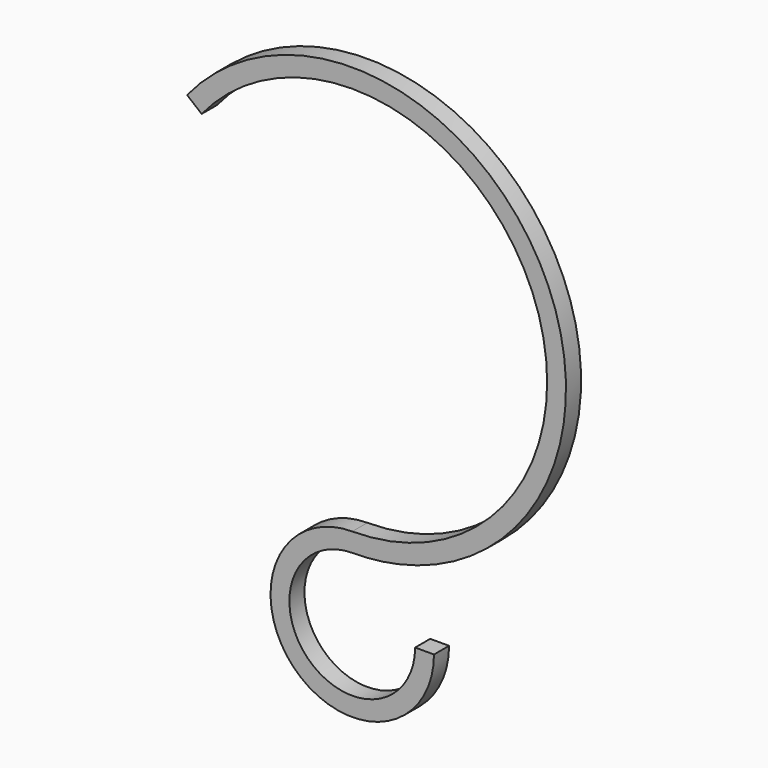
from build123d import *

# Parameters (mm, degrees)
F1_DEPTH = 3


with BuildPart() as f1:
    # F0 (on Front) → F1 (new body)
    with BuildSketch(Plane.XZ):
        with BuildLine():
            ThreePointArc((-23.9565223957, 19.6744767327), (10.4486316265, 29.1860599796), (31, 0))
            ThreePointArc((31, 0), (21.9203102168, -21.9203102168), (0, -31))
            ThreePointArc((0, -31), (3.7951823528, -31.5663122562), (7.2597095854, -33.2159090909))
            ThreePointArc((7.2597095854, -33.2159090909), (26.4842417855, -21.3209975622), (34, 0))
            ThreePointArc((34, 0), (11.4597895259, 32.010517397), (-26.2748955308, 21.578458352))
            Line((-26.2748955308, 21.578458352), (-23.9565223957, 19.6744767327))
        make_face()
        with BuildLine():
            ThreePointArc((7.2597095854, -33.2159090909), (3.7951823528, -31.5663122562), (0, -31))
            ThreePointArc((0, -31), (-3.7951823528, -31.5663122562), (-7.2597095854, -33.2159090909))
            ThreePointArc((-7.2597095854, -33.2159090909), (-3.6509650286, -33.8034089163), (-5.1e-08, -34))
            ThreePointArc((-5.1e-08, -34), (3.6509649778, -33.8034089217), (7.2597095854, -33.2159090909))
        make_face()
        with BuildLine():
            ThreePointArc((-5.1e-08, -34), (-3.6509650286, -33.8034089163), (-7.2597095854, -33.2159090909))
            ThreePointArc((-7.2597095854, -33.2159090909), (-6.1083457413, -55.4755440963), (13, -44))
            Line((13, -44), (10, -44))
            ThreePointArc((10, -44), (-7.0710677938, -51.0710678299), (-5.1e-08, -34))
        make_face()
    extrude(amount=F1_DEPTH)


solid = f1.part
